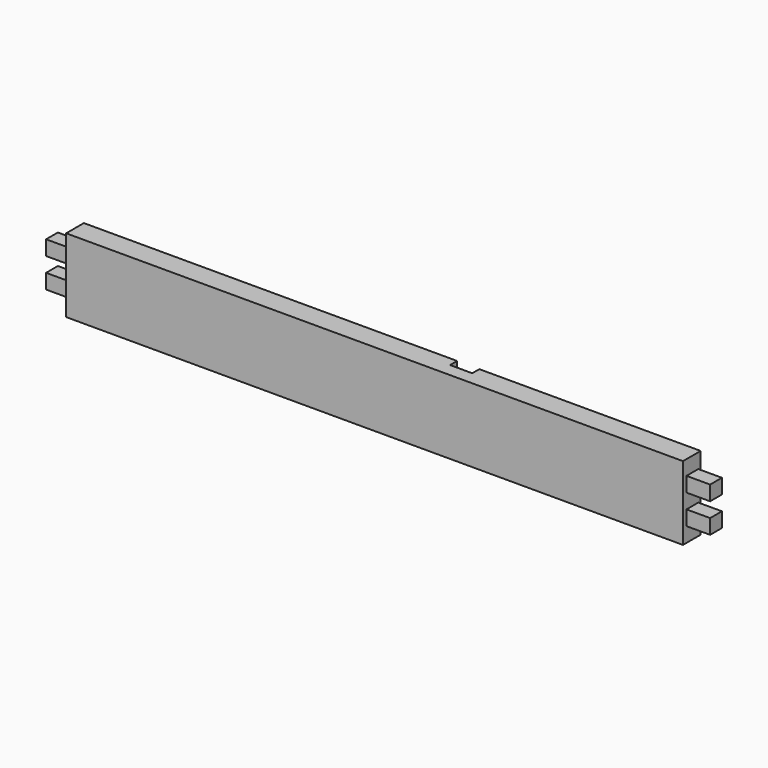
from build123d import *

# Parameters (mm, degrees)
F0_W     = 418
F0_H     = 50
F1_DEPTH = 15
F2_W     = 10
F2_H     = 10
F3_DEPTH = 16
F4_W     = 10
F4_H     = 10
F5_DEPTH = 16
F6_W     = 15
F6_H     = 30
F7_DEPTH = 6


# Not quite as in the source:
# - a feature names something its author has since deleted; it is built from what else it names


with BuildPart() as f1:
    # F0 (on Front) → F1 (new body)
    with BuildSketch(Plane.XZ):
        Rectangle(F0_W, F0_H)
    extrude(amount=F1_DEPTH)

    # F2 (on face) → F3 (join)
    with BuildSketch(Plane.YZ.offset(209)):
        with Locations((-7, 10)):
            Rectangle(F2_W, F2_H)
        with Locations((-7, -10)):
            Rectangle(F2_W, F2_H)
    extrude(amount=F3_DEPTH)

    # F4 (on face) → F5 (join)
    with BuildSketch(Plane(origin=(-209, 0, 0), x_dir=(0, -1, 0), z_dir=(-1, 0, 0))):
        with Locations((7, 10)):
            Rectangle(F4_W, F4_H)
        with Locations((7, -10)):
            Rectangle(F4_W, F4_H)
    extrude(amount=F5_DEPTH)

    # F6 (on face) → F7 (cut)
    with BuildSketch(Plane.XZ):
        with Locations((51.5, 10)):
            Rectangle(F6_W, F6_H)
    extrude(amount=F7_DEPTH, mode=Mode.SUBTRACT)


solid = f1.part
